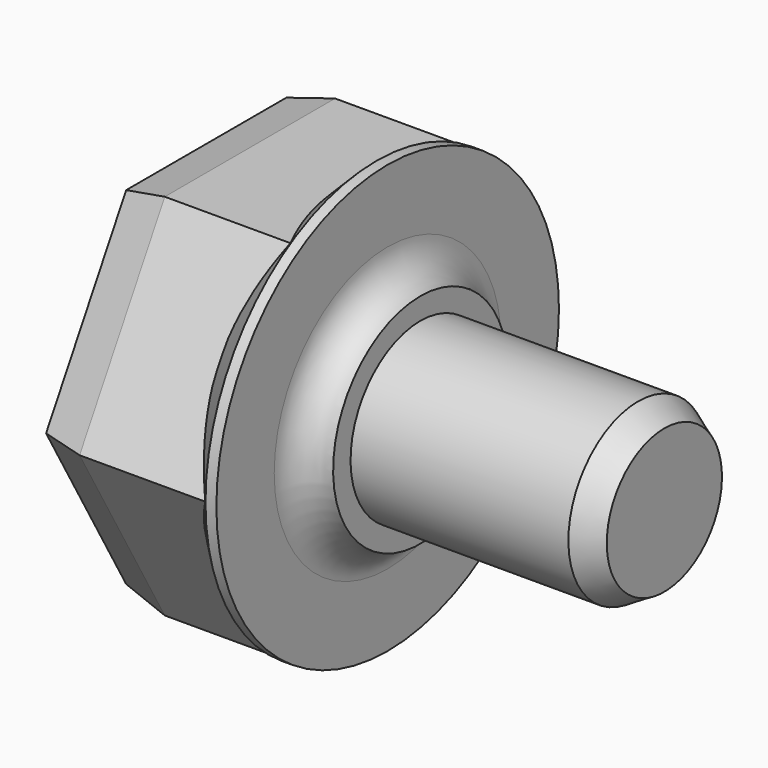
from build123d import *

# Parameters (mm, degrees)
F1_DEPTH = 8
F4_SIZE2 = 2
F4_SIZE  = 0.5
F5_SIZE2 = 0.7
F5_SIZE  = 1.2


# Not quite as in the source:
# - a feature names something its author has since deleted; it is built from what else it names


with BuildPart() as f1:
    # F0 (on Right) → F1 (new body)
    with BuildSketch(Plane.YZ):
        Polygon((4.8786097747, 8.45), (-4.8786097747, 8.45), (-9.7572195493, 0), (-4.8786097747, -8.45), (4.8786097747, -8.45), (9.7572195493, 0), align=None)
    extrude(amount=F1_DEPTH)

    # F2 (on Front) → F3 (revolve)
    with BuildSketch(Plane.XZ):
        with BuildLine():
            Line((8.315, 6.5), (8.315, 0))
            Line((8.315, 0), (21, 0))
            Line((21, 0), (21, 4))
            Line((21, 4), (9.815, 4))
            Line((9.815, 4), (9.815, 5))
            ThreePointArc((9.815, 5), (8.7543398282, 5.4393398282), (8.315, 6.5))
        make_face()
        Polygon((6.5, 8.5), (6.5, 0), (8.315, 0), (8.315, 6.5), (8.315, 9.815), (7.815, 9.815), align=None)
    revolve(axis=Axis((17.0378703874, 0, 0), (1, 0, 0)))

    # F4
    f4_edges = [f1.edges().sort_by_distance(p)[0] for p in [
        (0, 0, 8.45),
        (0, -7.317915, 4.225),
        (0, -7.317915, -4.225),
        (0, 0, -8.45),
        (0, 7.317915, -4.225),
        (0, 7.317915, 4.225),
    ]]
    f4_side = f1.faces().sort_by_distance((0, 0, 0))[0]
    chamfer(f4_edges, length=F4_SIZE, length2=F4_SIZE2, reference=f4_side)

    # F5
    f5_edges = [f1.edges().sort_by_distance(p)[0] for p in [
        (21, 0, -4),
    ]]
    f5_side = f1.faces().sort_by_distance((15.4075, 0, -4))[0]
    chamfer(f5_edges, length=F5_SIZE, length2=F5_SIZE2, reference=f5_side)


solid = f1.part
